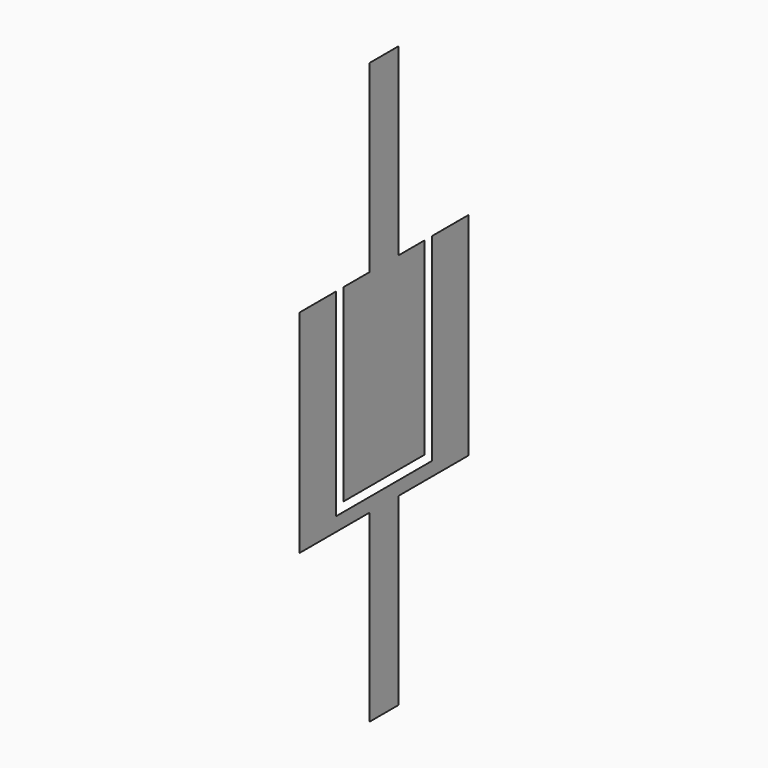
from build123d import *

# Parameters (mm, degrees)
F1_DEPTH = 0.0012


# Not quite as in the source:
# - a feature names something its author has since deleted; it is built from what else it names


with BuildPart() as f1:
    # F0 (on Right) → F1 (new body)
    with BuildSketch(Plane.YZ):
        Polygon((6.5217, 0), (0, 0), (0, -30), (12, -30), (12.39, -30), (12.39, -51.0653850647), (12.39, -56.0869), (17.61, -56.0869), (17.61, -30), (30, -30), (30, 0), (23.4783, 0), (23.4783, -28.04349), (7.82604, -28.04349), (6.5217, -28.04349), align=None)
    extrude(amount=F1_DEPTH)


with BuildPart() as f1b:
    # F0 (on Right) → F1, piece 2 (new body)
    with BuildSketch(Plane.YZ):
        Polygon((12.3913, 0), (11.4456, 0), (9, 0), (7.82604, 0), (7.82604, -26.73915), (22.17396, -26.73915), (22.17396, 0), (17.6113, 0), (17.6113, 26.0869), (12.3913, 26.0869), align=None)
    extrude(amount=F1_DEPTH)


solid = Compound([f1.part, f1b.part])
